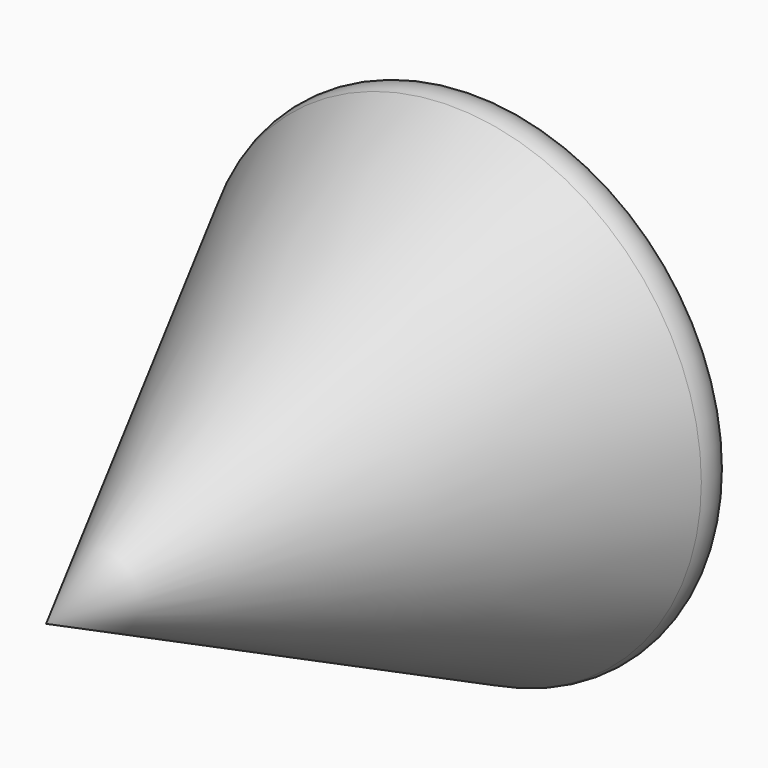
from build123d import *

# Parameters (mm, degrees)
F2_T = -2.54


# Not quite as in the source:
# - a fillet or chamfer that OpenCascade refuses, or shapes differently, is made with other operations: its cross-section is extruded or revolved along the edge and cut away or added


with BuildPart() as f1:
    # F0 (on Top) → F1 (revolve)
    with BuildSketch(Plane.XY):
        Polygon((0, 47.4987216294), (0, 44.8476299644), (0, -49.2661260068), (47.7196536958, 47.4987216294), align=None)
    revolve(axis=Axis((0, -2.2092480212, 0), (0, -1, 0)))

    # F2
    f2_openings = [f1.faces().sort_by_distance(p)[0] for p in [
        (0, 47.498722, 0),
    ]]
    offset(amount=F2_T, openings=f2_openings)

    # F3: fillet of radius 5.08 on 1 edges, made by hand

    # F3_s1 → F3_t2 (revolve, cut)
    with BuildSketch(Plane.XY):
        with BuildLine():
            ThreePointArc((45.2198112097, 42.4295968862), (45.7328319828, 45.0086691469), (44.8875848746, 47.4987216294))
            Line((44.8875848746, 47.4987216294), (47.7196536958, 47.4987216294))
            Line((47.7196536958, 47.4987216294), (45.2198112097, 42.4295968862))
        make_face()
    revolve(axis=Axis((0, 47.4987216294, 0), (0, -1, 0)), mode=Mode.SUBTRACT)


solid = f1.part
